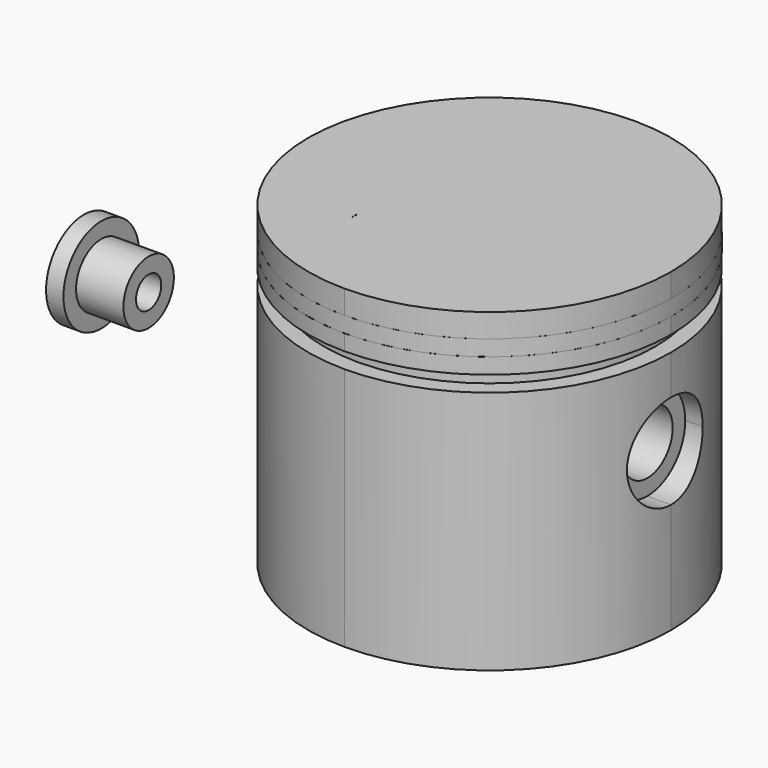
from build123d import *

# Parameters (mm, degrees)
F1_DEPTH  = 20
F2_DEPTH  = 18
F3_DEPTH  = 6
F5_DEPTH  = 12.5
F7_R      = 11.5
F7_R_2    = 10.5
F8_DEPTH  = 1
F10_R     = 11.5
F10_R_2   = 10.5
F11_DEPTH = 1
F12_DEPTH = 1
F13_R     = 3
F13_R_2   = 2
F14_DEPTH = 10


with BuildPart() as f1:
    # F0 (on Top) → F1 (new body)
    with BuildSketch(Plane.XY):
        with BuildLine():
            Line((0, 10.5), (0, 11.5))
            ThreePointArc((0, 11.5), (-8.1317279836, 8.1317279836), (-11.5, 0))
            Line((-11.5, 0), (-10.5, 0))
            ThreePointArc((-10.5, 0), (-7.4246212025, 7.4246212025), (0, 10.5))
        make_face()
        with BuildLine():
            Line((0, 9.5), (0, 10.5))
            ThreePointArc((0, 10.5), (-7.4246212025, 7.4246212025), (-10.5, 0))
            Line((-10.5, 0), (-4.4949756738, 0))
            Line((-4.4949756738, 0), (-4.499997726, 4.9954760621))
            ThreePointArc((-4.499997726, 4.9954760621), (-3.1835795671, 8.1803806596), (0, 9.5))
        make_face()
        with BuildLine():
            Line((-4.4949756738, 0), (0, 0))
            Line((0, 0), (0, 0.5))
            ThreePointArc((0, 0.5), (-3.1803806596, 1.8164204329), (-4.499997726, 4.9954760621))
            Line((-4.499997726, 4.9954760621), (-4.4949756738, 0))
        make_face()
        with BuildLine():
            Line((0, 0.5), (0, 9.5))
            ThreePointArc((0, 9.5), (-3.1835795671, 8.1803806596), (-4.499997726, 4.9954760621))
            ThreePointArc((-4.499997726, 4.9954760621), (-3.1803806596, 1.8164204329), (0, 0.5))
        make_face()
        with BuildLine():
            ThreePointArc((4.5, 5), (3.1819805153, 8.1819805153), (0, 9.5))
            Line((0, 9.5), (0, 0.5))
            ThreePointArc((0, 0.5), (3.1819805153, 1.8180194847), (4.5, 5))
        make_face()
        with BuildLine():
            Line((10.5, 0), (11.5, 0))
            ThreePointArc((11.5, 0), (8.1317279836, 8.1317279836), (0, 11.5))
            Line((0, 11.5), (0, 10.5))
            ThreePointArc((0, 10.5), (7.4246212025, 7.4246212025), (10.5, 0))
        make_face()
        with BuildLine():
            Line((4.5, -5), (4.5, 0))
            Line((4.5, 0), (0, 0))
            Line((0, 0), (0, -0.5))
            ThreePointArc((0, -0.5), (3.1819805153, -1.8180194847), (4.5, -5))
        make_face()
        with BuildLine():
            ThreePointArc((0, -10.5), (7.4246212025, -7.4246212025), (10.5, 0))
            Line((10.5, 0), (4.5, 0))
            Line((4.5, 0), (4.5, -5))
            ThreePointArc((4.5, -5), (3.1819805153, -8.1819805153), (0, -9.5))
            Line((0, -9.5), (0, -10.5))
        make_face()
        with BuildLine():
            ThreePointArc((-11.5, 0), (-8.1317279836, -8.1317279836), (0, -11.5))
            Line((0, -11.5), (0, -10.5))
            ThreePointArc((0, -10.5), (-7.4246212025, -7.4246212025), (-10.5, 0))
            Line((-10.5, 0), (-11.5, 0))
        make_face()
        with BuildLine():
            ThreePointArc((-10.5, 0), (-7.4246212025, -7.4246212025), (0, -10.5))
            Line((0, -10.5), (0, -9.5))
            ThreePointArc((0, -9.5), (-3.0722026892, -8.28809529), (-4.4896423078, -5.3051425051))
            ThreePointArc((-4.4896423078, -5.3051425051), (-4.499997726, -5.0045239379), (-4.4902467638, -4.7038851573))
            Line((-4.4902467638, -4.7038851573), (-4.4949756738, 0))
            Line((-4.4949756738, 0), (-10.5, 0))
        make_face()
        with BuildLine():
            Line((0, -0.5), (0, 0))
            Line((0, 0), (-4.4949756738, 0))
            Line((-4.4949756738, 0), (-4.4902467638, -4.7038851573))
            ThreePointArc((-4.4902467638, -4.7038851573), (-3.0755067231, -1.7149949169), (0, -0.5))
        make_face()
        with BuildLine():
            ThreePointArc((-4.4896423078, -5.3051425051), (-3.0722026892, -8.28809529), (0, -9.5))
            Line((0, -9.5), (0, -0.5))
            ThreePointArc((0, -0.5), (-3.0755067231, -1.7149949169), (-4.4902467638, -4.7038851573))
            Line((-4.4902467638, -4.7038851573), (-4.4896423078, -5.3051425051))
        make_face()
        with BuildLine():
            Line((0, -0.5), (0, -9.5))
            ThreePointArc((0, -9.5), (3.1819805153, -8.1819805153), (4.5, -5))
            ThreePointArc((4.5, -5), (3.1819805153, -1.8180194847), (0, -0.5))
        make_face()
        with BuildLine():
            ThreePointArc((0, -11.5), (8.1317279836, -8.1317279836), (11.5, 0))
            Line((11.5, 0), (10.5, 0))
            ThreePointArc((10.5, 0), (7.4246212025, -7.4246212025), (0, -10.5))
            Line((0, -10.5), (0, -11.5))
        make_face()
        with BuildLine():
            Line((4.5, 0), (10.5, 0))
            ThreePointArc((10.5, 0), (7.4246212025, 7.4246212025), (0, 10.5))
            Line((0, 10.5), (0, 9.5))
            ThreePointArc((0, 9.5), (3.1819805153, 8.1819805153), (4.5, 5))
            Line((4.5, 5), (4.5, 0))
        make_face()
        with BuildLine():
            Line((0, 0), (4.5, 0))
            Line((4.5, 0), (4.5, 5))
            ThreePointArc((4.5, 5), (3.1819805153, 1.8180194847), (0, 0.5))
            Line((0, 0.5), (0, 0))
        make_face()
    extrude(amount=F1_DEPTH)

    # F0 (on Top) → F2 (cut)
    with BuildSketch(Plane.XY):
        with BuildLine():
            ThreePointArc((-4.4896423078, -5.3051425051), (-3.0722026892, -8.28809529), (0, -9.5))
            Line((0, -9.5), (0, -0.5))
            ThreePointArc((0, -0.5), (-3.0755067231, -1.7149949169), (-4.4902467638, -4.7038851573))
            Line((-4.4902467638, -4.7038851573), (-4.4896423078, -5.3051425051))
        make_face()
        with BuildLine():
            Line((0, -0.5), (0, -9.5))
            ThreePointArc((0, -9.5), (3.1819805153, -8.1819805153), (4.5, -5))
            ThreePointArc((4.5, -5), (3.1819805153, -1.8180194847), (0, -0.5))
        make_face()
        with BuildLine():
            Line((4.5, -5), (4.5, 0))
            Line((4.5, 0), (0, 0))
            Line((0, 0), (0, -0.5))
            ThreePointArc((0, -0.5), (3.1819805153, -1.8180194847), (4.5, -5))
        make_face()
        with BuildLine():
            Line((0, 0), (4.5, 0))
            Line((4.5, 0), (4.5, 5))
            ThreePointArc((4.5, 5), (3.1819805153, 1.8180194847), (0, 0.5))
            Line((0, 0.5), (0, 0))
        make_face()
        with BuildLine():
            ThreePointArc((4.5, 5), (3.1819805153, 8.1819805153), (0, 9.5))
            Line((0, 9.5), (0, 0.5))
            ThreePointArc((0, 0.5), (3.1819805153, 1.8180194847), (4.5, 5))
        make_face()
        with BuildLine():
            Line((0, 0.5), (0, 9.5))
            ThreePointArc((0, 9.5), (-3.1835795671, 8.1803806596), (-4.499997726, 4.9954760621))
            ThreePointArc((-4.499997726, 4.9954760621), (-3.1803806596, 1.8164204329), (0, 0.5))
        make_face()
        with BuildLine():
            Line((0, -0.5), (0, 0))
            Line((0, 0), (-4.4949756738, 0))
            Line((-4.4949756738, 0), (-4.4902467638, -4.7038851573))
            ThreePointArc((-4.4902467638, -4.7038851573), (-3.0755067231, -1.7149949169), (0, -0.5))
        make_face()
        with BuildLine():
            Line((-4.4949756738, 0), (0, 0))
            Line((0, 0), (0, 0.5))
            ThreePointArc((0, 0.5), (-3.1803806596, 1.8164204329), (-4.499997726, 4.9954760621))
            Line((-4.499997726, 4.9954760621), (-4.4949756738, 0))
        make_face()
    extrude(amount=F2_DEPTH, mode=Mode.SUBTRACT)

    # F0 (on Top) → F3 (cut)
    with BuildSketch(Plane.XY):
        with BuildLine():
            ThreePointArc((-10.5, 0), (-7.4246212025, -7.4246212025), (0, -10.5))
            Line((0, -10.5), (0, -9.5))
            ThreePointArc((0, -9.5), (-3.0722026892, -8.28809529), (-4.4896423078, -5.3051425051))
            ThreePointArc((-4.4896423078, -5.3051425051), (-4.499997726, -5.0045239379), (-4.4902467638, -4.7038851573))
            Line((-4.4902467638, -4.7038851573), (-4.4949756738, 0))
            Line((-4.4949756738, 0), (-10.5, 0))
        make_face()
        with BuildLine():
            ThreePointArc((0, -10.5), (7.4246212025, -7.4246212025), (10.5, 0))
            Line((10.5, 0), (4.5, 0))
            Line((4.5, 0), (4.5, -5))
            ThreePointArc((4.5, -5), (3.1819805153, -8.1819805153), (0, -9.5))
            Line((0, -9.5), (0, -10.5))
        make_face()
        with BuildLine():
            Line((4.5, 0), (10.5, 0))
            ThreePointArc((10.5, 0), (7.4246212025, 7.4246212025), (0, 10.5))
            Line((0, 10.5), (0, 9.5))
            ThreePointArc((0, 9.5), (3.1819805153, 8.1819805153), (4.5, 5))
            Line((4.5, 5), (4.5, 0))
        make_face()
        with BuildLine():
            Line((0, 9.5), (0, 10.5))
            ThreePointArc((0, 10.5), (-7.4246212025, 7.4246212025), (-10.5, 0))
            Line((-10.5, 0), (-4.4949756738, 0))
            Line((-4.4949756738, 0), (-4.499997726, 4.9954760621))
            ThreePointArc((-4.499997726, 4.9954760621), (-3.1835795671, 8.1803806596), (0, 9.5))
        make_face()
    extrude(amount=F3_DEPTH, mode=Mode.SUBTRACT)

    # F4 (on Right) → F5 (cut, symmetric)
    with BuildSketch(Plane.YZ):
        with BuildLine():
            ThreePointArc((3, 10), (2.1213203436, 12.1213203436), (0, 13))
            Line((0, 13), (0, 7))
            ThreePointArc((0, 7), (2.1213203436, 7.8786796564), (3, 10))
        make_face()
        with BuildLine():
            Line((0, 7), (0, 13))
            ThreePointArc((0, 13), (-3, 10), (0, 7))
        make_face()
    extrude(amount=F5_DEPTH, both=True, mode=Mode.SUBTRACT)

    # F7 (on offset) → F8 (cut)
    with BuildSketch(Plane.XY.offset(18.5)):
        Circle(F7_R)
        Circle(F7_R_2, mode=Mode.SUBTRACT)
    extrude(amount=-F8_DEPTH, mode=Mode.SUBTRACT)

    # F10 (on offset) → F11 (cut)
    with BuildSketch(Plane.XY.offset(16.5)):
        Circle(F10_R)
        Circle(F10_R_2, mode=Mode.SUBTRACT)
    extrude(amount=-F11_DEPTH, mode=Mode.SUBTRACT)


with BuildPart() as f12:
    # F7 (on offset) → F12 (new body)
    with BuildSketch(Plane.XY.offset(18.5)):
        Circle(F7_R)
        Circle(F7_R_2, mode=Mode.SUBTRACT)
    extrude(amount=-F12_DEPTH)


with BuildPart() as f14:
    # F13 (on face) → F14 (new body, symmetric)
    with BuildSketch(Plane.YZ):
        with Locations((0, 10)):
            Circle(F13_R)
        with Locations((0, 10)):
            Circle(F13_R_2, mode=Mode.SUBTRACT)
    extrude(amount=F14_DEPTH, both=True)


with BuildPart() as f16:
    # F15 (on Front) → F16 (revolve)
    with BuildSketch(Plane.XZ):
        with BuildLine():
            Line((-26.0740043477, 9.0888299271), (-21.6175651103, 9.0888299271))
            Line((-21.6175651103, 9.0888299271), (-21.6175651103, 10.0888299271))
            Line((-21.6175651103, 10.0888299271), (-24.6175651103, 10.0888299271))
            Line((-24.6175651103, 10.0888299271), (-24.6175651103, 11.0888299271))
            Line((-24.6175651103, 11.0888299271), (-25.7193667659, 11.0888299271))
            ThreePointArc((-25.7193667659, 11.0888299271), (-25.940928482, 10.0966750291), (-26.0740043477, 9.0888299271))
        make_face()
    revolve(axis=Axis((-20.3675651103, 0, 8.0888299271), (1, 0, 0)))


solid = Compound([f1.part, f12.part, f14.part, f16.part])
